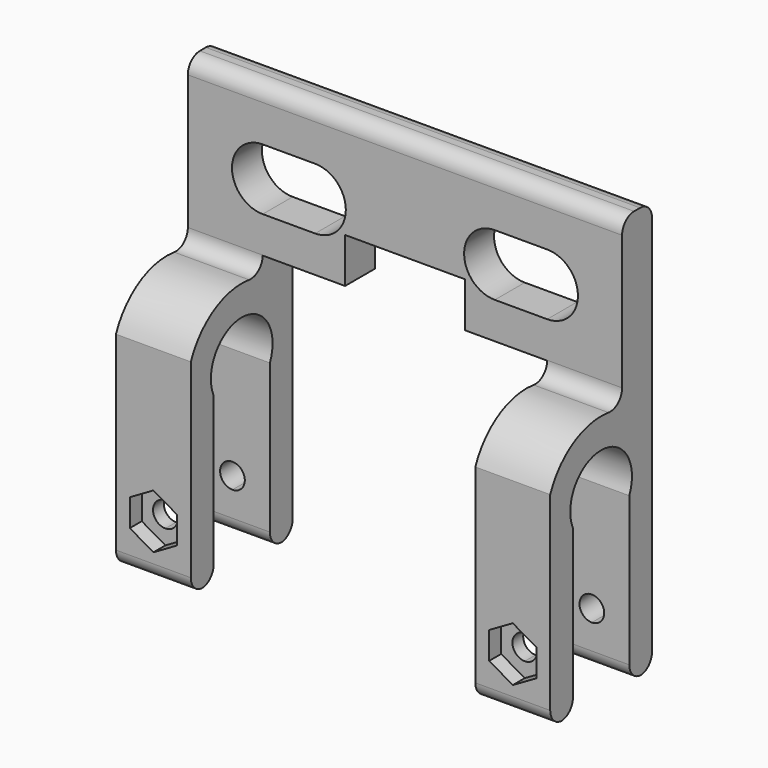
from build123d import *

# Parameters (mm, degrees)
F1_DEPTH     = 17
F3_DEPTH     = 80
F4_T4_DEPTH  = 16.4862536334
F4_T10_DEPTH = 10
F4_T15_DEPTH = 10
F4_T20_DEPTH = 10
F4_T25_DEPTH = 10
F4_T30_DEPTH = 16.4862536334
F4_T33_DEPTH = 68
F4_T35_DEPTH = 20
F4_T37_DEPTH = 20
F5_R         = 1.65
F6_DEPTH     = 2


# Not quite as in the source:
# - a fillet or chamfer that OpenCascade refuses, or shapes differently, is made with other operations: its cross-section is extruded or revolved along the edge and cut away or added


with BuildPart() as f1:
    # F0 (on Front) → F1 (new body)
    with BuildSketch(Plane.XZ):
        Polygon((-13, 18.9721025527), (-13, -25), (-8, -25), (-3, -25), (-3, -5), (-3, 0), (-3, 5), (-3, 10), (8, 10), (8, 16), (24, 16), (24, 10), (35, 10), (35, 5), (35, 0), (35, -5), (35, -25), (40, -25), (45, -25), (45, 25), (45, 30), (-13, 30), (-13, 25), align=None)
        Polygon((-4.9, -19.7897858345), (-8, -21.579571669), (-11.1, -19.7897858345), (-11.1, -16.2102141655), (-8, -14.420428331), (-4.9, -16.2102141655), align=None, mode=Mode.SUBTRACT)
        Polygon((43.1, -19.7897858345), (40, -21.579571669), (36.9, -19.7897858345), (36.9, -16.2102141655), (40, -14.420428331), (43.1, -16.2102141655), align=None, mode=Mode.SUBTRACT)
        with BuildLine():
            ThreePointArc((-3, 14.8721025527), (-7.1, 18.9721025527), (-3, 23.0721025527))
            Line((-3, 23.0721025527), (4, 23.0721025527))
            ThreePointArc((4, 23.0721025527), (8.1, 18.9721025527), (4, 14.8721025527))
            Line((4, 14.8721025527), (-3, 14.8721025527))
        make_face(mode=Mode.SUBTRACT)
        with BuildLine():
            ThreePointArc((28, 14.8721025527), (23.9, 18.9721025527), (28, 23.0721025527))
            Line((28, 23.0721025527), (35, 23.0721025527))
            ThreePointArc((35, 23.0721025527), (39.1, 18.9721025527), (35, 14.8721025527))
            Line((35, 14.8721025527), (28, 14.8721025527))
        make_face(mode=Mode.SUBTRACT)
        Polygon((36.9, -19.7897858345), (40, -21.579571669), (43.1, -19.7897858345), (43.1, -16.2102141655), (40, -14.420428331), (36.9, -16.2102141655), align=None)
        with BuildLine():
            ThreePointArc((41.65, -18), (41.166726189, -19.166726189), (40, -19.65))
            ThreePointArc((40, -19.65), (38.833273811, -16.833273811), (41.65, -18))
        make_face(mode=Mode.SUBTRACT)
        Polygon((-11.1, -19.7897858345), (-8, -21.579571669), (-4.9, -19.7897858345), (-4.9, -16.2102141655), (-8, -14.420428331), (-11.1, -16.2102141655), align=None)
        with BuildLine():
            ThreePointArc((-6.35, -18), (-6.833273811, -19.166726189), (-8, -19.65))
            ThreePointArc((-8, -19.65), (-9.166726189, -16.833273811), (-6.35, -18))
        make_face(mode=Mode.SUBTRACT)
    extrude(amount=F1_DEPTH)

    # F2 (on face) → F3 (cut)
    with BuildSketch(Plane.YZ.offset(45)):
        with BuildLine():
            Line((-17, 30), (-17, 2.3871079109))
            ThreePointArc((-17, 2.3871079109), (-12.0593125845, 7.429341251), (-5, 7.4541409972))
            Line((-5, 7.4541409972), (-5, 30))
            Line((-5, 30), (-17, 30))
        make_face()
        with BuildLine():
            Line((-3.8, -25), (-3.8, -3.1053503271))
            ThreePointArc((-3.8, -3.1053503271), (-8.5, 4.15), (-13.2, -3.1053503271))
            Line((-13.2, -3.1053503271), (-13.2, -25))
            Line((-13.2, -25), (-4, -25))
            Line((-4, -25), (-3.8, -25))
        make_face()
    extrude(amount=-F3_DEPTH, mode=Mode.SUBTRACT)

    # F4: fillet of radius 2 on 12 edges, made by hand


with BuildPart() as f4_tool2:
    # F4_s3 → F4_t4 (new body)
    with BuildSketch(Plane.YZ.offset(3.4862536334)):
        with BuildLine():
            ThreePointArc((-5, 10.0486424505), (-5.6843474227, 8.5423030811), (-7.269058296, 8.0668231769))
            ThreePointArc((-7.269058296, 8.0668231769), (-6.1147752276, 7.8336404039), (-5, 7.4541409972))
            Line((-5, 7.4541409972), (-5, 10.0486424505))
        make_face()
    extrude(amount=-F4_T4_DEPTH)

    split(bisect_by=Plane.YZ.offset(-3), keep=Keep.TOP)

    split(bisect_by=Plane.XY.offset(10), keep=Keep.TOP)


with BuildPart() as f1_1:
    add(f1.part)

    # F4_t1: union F4_tool2
    add(f4_tool2.part)


with BuildPart() as f4_tool8:
    # F4_s9 → F4_t10 (new body)
    with BuildSketch(Plane.YZ.offset(-3)):
        with BuildLine():
            ThreePointArc((-5, 10.0486424505), (-5.6843474227, 8.5423030811), (-7.269058296, 8.0668231769))
            ThreePointArc((-7.269058296, 8.0668231769), (-6.1147752276, 7.8336404039), (-5, 7.4541409972))
            Line((-5, 7.4541409972), (-5, 10.0486424505))
        make_face()
    extrude(amount=-F4_T10_DEPTH)

    split(bisect_by=Plane.XY.offset(10), keep=Keep.TOP)


with BuildPart() as f1_2:
    add(f1_1.part)

    # F4_t7: union F4_tool8
    add(f4_tool8.part)


with BuildPart() as f4_tool13:
    # F4_s14 → F4_t15 (new body)
    with BuildSketch(Plane.YZ.offset(-3)):
        with BuildLine():
            ThreePointArc((-5, 10.0486424505), (-5.6843474227, 8.5423030811), (-7.269058296, 8.0668231769))
            ThreePointArc((-7.269058296, 8.0668231769), (-6.1147752276, 7.8336404039), (-5, 7.4541409972))
            Line((-5, 7.4541409972), (-5, 10.0486424505))
        make_face()
    extrude(amount=-F4_T15_DEPTH)

    split(bisect_by=Plane.XY.offset(10), keep=Keep.BOTTOM)


with BuildPart() as f1_3:
    add(f1_2.part)

    # F4_t12: union F4_tool13
    add(f4_tool13.part)


with BuildPart() as f4_tool18:
    # F4_s19 → F4_t20 (new body)
    with BuildSketch(Plane.YZ.offset(45)):
        with BuildLine():
            ThreePointArc((-5, 10.0486424505), (-5.6843474227, 8.5423030811), (-7.269058296, 8.0668231769))
            ThreePointArc((-7.269058296, 8.0668231769), (-6.1147752276, 7.8336404039), (-5, 7.4541409972))
            Line((-5, 7.4541409972), (-5, 10.0486424505))
        make_face()
    extrude(amount=-F4_T20_DEPTH)

    split(bisect_by=Plane.XY.offset(10), keep=Keep.TOP)


with BuildPart() as f1_4:
    add(f1_3.part)

    # F4_t17: union F4_tool18
    add(f4_tool18.part)


with BuildPart() as f4_tool23:
    # F4_s24 → F4_t25 (new body)
    with BuildSketch(Plane.YZ.offset(45)):
        with BuildLine():
            ThreePointArc((-5, 10.0486424505), (-5.6843474227, 8.5423030811), (-7.269058296, 8.0668231769))
            ThreePointArc((-7.269058296, 8.0668231769), (-6.1147752276, 7.8336404039), (-5, 7.4541409972))
            Line((-5, 7.4541409972), (-5, 10.0486424505))
        make_face()
    extrude(amount=-F4_T25_DEPTH)

    split(bisect_by=Plane.XY.offset(10), keep=Keep.BOTTOM)


with BuildPart() as f1_5:
    add(f1_4.part)

    # F4_t22: union F4_tool23
    add(f4_tool23.part)


with BuildPart() as f4_tool28:
    # F4_s29 → F4_t30 (new body)
    with BuildSketch(Plane.YZ.offset(45)):
        with BuildLine():
            ThreePointArc((-5, 10.0486424505), (-5.6843474227, 8.5423030811), (-7.269058296, 8.0668231769))
            ThreePointArc((-7.269058296, 8.0668231769), (-6.1147752276, 7.8336404039), (-5, 7.4541409972))
            Line((-5, 7.4541409972), (-5, 10.0486424505))
        make_face()
    extrude(amount=-F4_T30_DEPTH)

    split(bisect_by=Plane.XY.offset(10), keep=Keep.TOP)

    split(bisect_by=Plane.YZ.offset(35), keep=Keep.BOTTOM)


with BuildPart() as f1_6:
    add(f1_5.part)

    # F4_t27: union F4_tool28
    add(f4_tool28.part)

    # F4_s34 → F4_t33 (cut)
    with BuildSketch(Plane.YZ.offset(-18)):
        with BuildLine():
            ThreePointArc((-5, 28), (-4.4142135624, 29.4142135624), (-3, 30))
            Line((-3, 30), (-5, 30))
            Line((-5, 30), (-5, 28))
        make_face()
        with BuildLine():
            ThreePointArc((-2, 30), (-0.5857864376, 29.4142135624), (0, 28))
            Line((0, 28), (0, 30))
            Line((0, 30), (-2, 30))
        make_face()
    extrude(amount=F4_T33_DEPTH, mode=Mode.SUBTRACT)

    # F4_s36 → F4_t35 (cut)
    with BuildSketch(Plane.YZ.offset(30)):
        with BuildLine():
            ThreePointArc((-15, -25), (-16.4142135624, -24.4142135624), (-17, -23))
            Line((-17, -23), (-17, -25))
            Line((-17, -25), (-15, -25))
        make_face()
        with BuildLine():
            ThreePointArc((-13.2, -23), (-13.7857864376, -24.4142135624), (-15.2, -25))
            Line((-15.2, -25), (-13.2, -25))
            Line((-13.2, -25), (-13.2, -23))
        make_face()
        with BuildLine():
            ThreePointArc((-1.8, -25), (-3.2142135624, -24.4142135624), (-3.8, -23))
            Line((-3.8, -23), (-3.8, -25))
            Line((-3.8, -25), (-1.8, -25))
        make_face()
        with BuildLine():
            ThreePointArc((-2, -25), (-0.5857864376, -24.4142135624), (0, -23))
            Line((0, -23), (0, -25))
            Line((0, -25), (-2, -25))
        make_face()
    extrude(amount=F4_T35_DEPTH, mode=Mode.SUBTRACT)

    # F4_s38 → F4_t37 (cut)
    with BuildSketch(Plane.YZ.offset(-18)):
        with BuildLine():
            ThreePointArc((-15, -25), (-16.4142135624, -24.4142135624), (-17, -23))
            Line((-17, -23), (-17, -25))
            Line((-17, -25), (-15, -25))
        make_face()
        with BuildLine():
            ThreePointArc((-13.2, -23), (-13.7857864376, -24.4142135624), (-15.2, -25))
            Line((-15.2, -25), (-13.2, -25))
            Line((-13.2, -25), (-13.2, -23))
        make_face()
        with BuildLine():
            ThreePointArc((-1.8, -25), (-3.2142135624, -24.4142135624), (-3.8, -23))
            Line((-3.8, -23), (-3.8, -25))
            Line((-3.8, -25), (-1.8, -25))
        make_face()
        with BuildLine():
            ThreePointArc((-2, -25), (-0.5857864376, -24.4142135624), (0, -23))
            Line((0, -23), (0, -25))
            Line((0, -25), (-2, -25))
        make_face()
    extrude(amount=F4_T37_DEPTH, mode=Mode.SUBTRACT)

    # F5 (on face) → F6 (cut)
    with BuildSketch(Plane.XZ.offset(17)):
        Polygon((-4.85, -19.8186533479), (-4.85, -16.1813466521), (-8, -14.3626933041), (-11.15, -16.1813466521), (-11.15, -19.8186533479), (-8, -21.6373066959), align=None)
        with Locations((-8, -18)):
            Circle(F5_R, mode=Mode.SUBTRACT)
        Polygon((36.85, -16.1813466521), (36.85, -19.8186533479), (40, -21.6373066959), (43.15, -19.8186533479), (43.15, -16.1813466521), (40, -14.3626933041), align=None)
    extrude(amount=-F6_DEPTH, mode=Mode.SUBTRACT)


solid = f1_6.part
